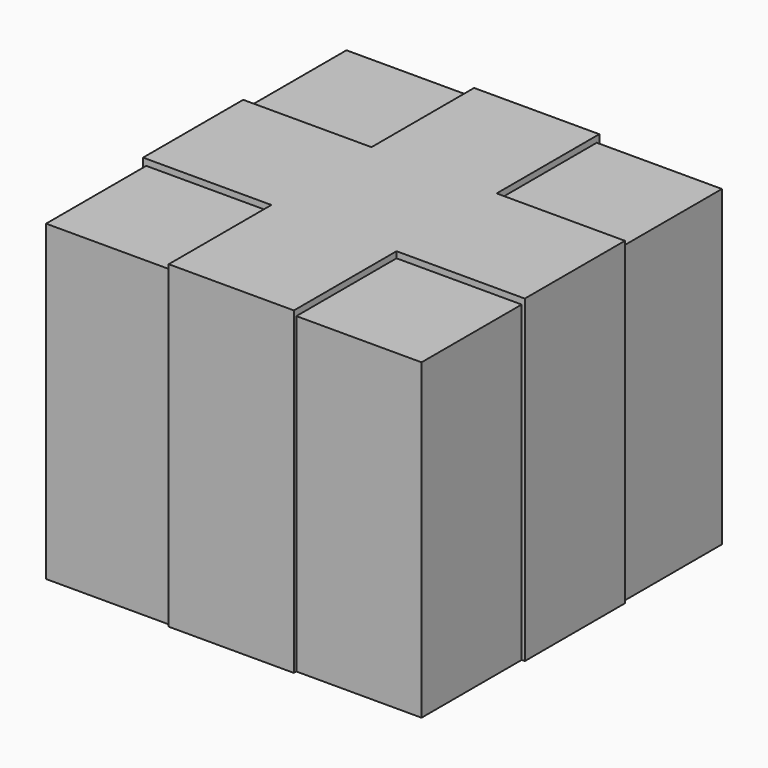
from build123d import *

# Parameters (mm, degrees)
F0_W     = 50.8
F0_H     = 1.27
F1_DEPTH = 127
F0_W_2   = 1.27
F0_H_2   = 50.8
F2_DEPTH = 129.54
F3_DEPTH = 152.4
F4_DEPTH = 152.4


with BuildPart() as f1:
    # F0 (on Top) → F1 (new body)
    with BuildSketch(Plane.XY):
        Polygon((-25.4, 76.2), (-76.2, 76.2), (-76.2, 25.4), (-76.2, -25.4), (-76.2, -76.2), (-25.4, -76.2), (25.4, -76.2), (76.2, -76.2), (76.2, -25.4), (76.2, 25.4), (76.2, 76.2), (25.4, 76.2), (25.4, 74.93), (-25.4, 74.93), align=None)
        with Locations((0, 75.565)):
            Rectangle(F0_W, F0_H)
    extrude(amount=F1_DEPTH)


with BuildPart() as f2:
    # F0 (on Top) → F2 (new body)
    with BuildSketch(Plane.XY):
        with Locations((76.835, 0)):
            Rectangle(F0_W_2, F0_H_2)
    extrude(amount=F2_DEPTH)

    # F4 (add): a face of the model
    f4_faces = [f2.faces().sort_by_distance(p)[0] for p in [
        (76.2, 0, 64.77),
    ]]


with BuildPart() as f2b:
    # F0 (on Top) → F2, piece 2 (new body)
    with BuildSketch(Plane.XY):
        with Locations((0, 76.835)):
            Rectangle(F0_W, F0_H)
    extrude(amount=F2_DEPTH)

    # F3 (add): a face of the model
    f3_faces = [f2b.faces().sort_by_distance(p)[0] for p in [
        (0, 76.2, 64.77),
    ]]


with BuildPart() as f2c:
    # F0 (on Top) → F2, piece 3 (new body)
    with BuildSketch(Plane.XY):
        with Locations((0, -76.835)):
            Rectangle(F0_W, F0_H)
    extrude(amount=F2_DEPTH)


with BuildPart() as f2d:
    # F0 (on Top) → F2, piece 4 (new body)
    with BuildSketch(Plane.XY):
        with Locations((-76.835, 0)):
            Rectangle(F0_W_2, F0_H_2)
    extrude(amount=F2_DEPTH)


with BuildPart() as f2b_1:
    add(f2b.part)

    add(f2c.part)  # F3 merges F2c
    extrude(f3_faces, amount=F3_DEPTH)


with BuildPart() as f2_1:
    add(f2.part)

    add(f2b_1.part)  # F4 merges F2b

    add(f2d.part)  # F4 merges F2d
    extrude(f4_faces, amount=F4_DEPTH)


solid = Compound([f1.part, f2_1.part])
